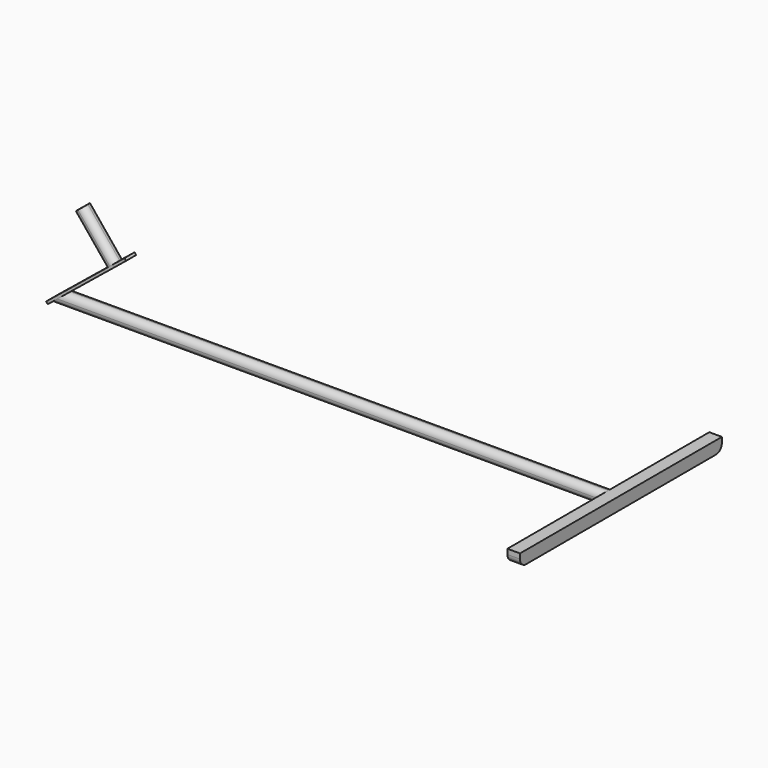
from build123d import *

# Parameters (mm, degrees)
F0_W      = 254
F0_H      = 12.7
F1_DEPTH  = 12.7
F3_DEPTH  = 558.8
F4_R      = 7.62
F6_DEPTH  = 12.7
F7_W      = 101.6
F7_H      = 12.7
F8_DEPTH  = 2.54
F10_DEPTH = 50.8


with BuildPart() as f1:
    # F0 (on Right) → F1 (new body)
    with BuildSketch(Plane.YZ):
        Rectangle(F0_W, F0_H)
    extrude(amount=F1_DEPTH)

    # F2 (on face) → F3 (join)
    with BuildSketch(Plane(origin=(0, 0, 0), x_dir=(0, -1, 0), z_dir=(-1, 0, 0))):
        with BuildLine():
            ThreePointArc((-6.84e-08, -6.35), (4.4901280364, -4.4901280847), (6.35, 0))
            ThreePointArc((6.35, 0), (4.4901280521, 4.4901280689), (-2.37e-08, 6.35))
            ThreePointArc((-2.37e-08, 6.35), (-6.35, 2.23e-08), (-6.84e-08, -6.35))
        make_face()
    extrude(amount=F3_DEPTH)

    # F4
    f4_edges = [f1.edges().sort_by_distance(p)[0] for p in [
        (6.35, -127, -6.35),
        (6.35, 127, -6.35),
    ]]
    fillet(f4_edges, radius=F4_R)

    # F5 (on Front) → F6 (cut, symmetric)
    with BuildSketch(Plane.XZ):
        Polygon((-541.0905659676, 6.7056384869), (-558.8, 6.7056384869), (-558.8, -7.6832813211), align=None)
    extrude(amount=F6_DEPTH, both=True, mode=Mode.SUBTRACT)

    # F7 (on face) → F8 (join)
    with BuildSketch(Plane(origin=(-218.4449745832, 0, 268.8552663249), x_dir=(0.7761139002, 0, 0.630592748), z_dir=(-0.630592748, 0, 0.7761139002))):
        with Locations((-388.1941093914, 0)):
            Rectangle(F7_W, F7_H)
    extrude(amount=F8_DEPTH)

    # F9 (on face) → F10 (join)
    with BuildSketch(Plane(origin=(-220.0466801631, 0, 270.8265956315), x_dir=(0.7761139002, 0, 0.630592748), z_dir=(-0.630592748, 0, 0.7761139002))):
        with BuildLine():
            ThreePointArc((-356.4441093914, -6.35), (-351.9539813308, -4.4901280605), (-350.0941093914, 0))
            ThreePointArc((-350.0941093914, 0), (-351.9539813308, 4.4901280605), (-356.4441093914, 6.35))
            ThreePointArc((-356.4441093914, 6.35), (-362.7941093914, 0), (-356.4441093914, -6.35))
        make_face()
    extrude(amount=F10_DEPTH)


solid = f1.part
